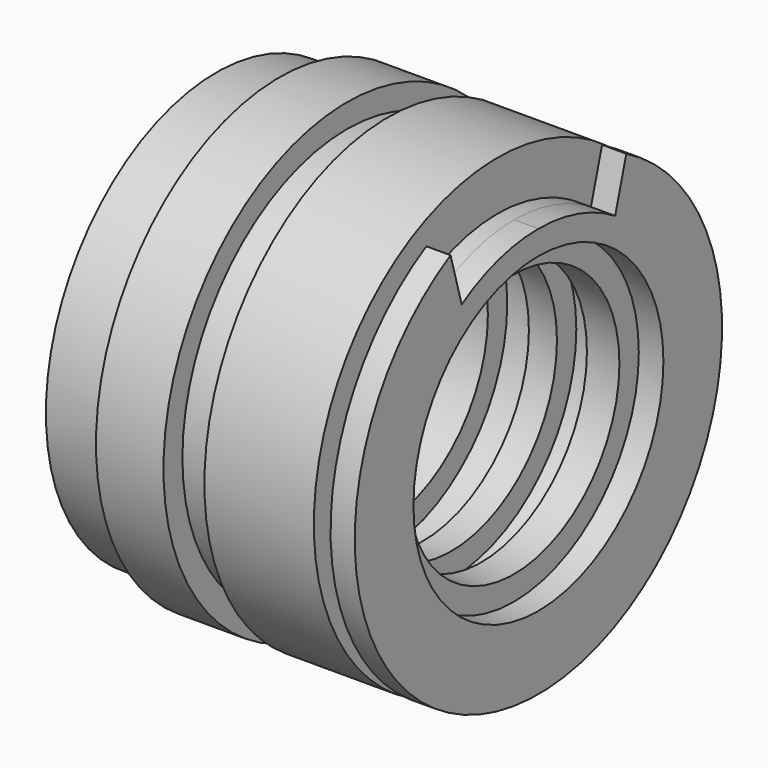
from build123d import *

# Parameters (mm, degrees)
F3_DEPTH = 4.6736


# Not quite as in the source:
# - after a boolean that leaves OpenCascade's solid faulty, fix() repairs it


with BuildPart() as f1:
    # F0 (on Top) → F1 (revolve)
    with BuildSketch(Plane.XY):
        Polygon((-4.7498, 30.1625), (0, 30.1625), (0, 44.323), (-4.6736, 44.323), (-4.6736, 34.798), (-7.8994, 34.798), (-7.8994, 44.323), (-29.0322, 44.323), (-29.0322, 39.751), (-36.9316, 39.751), (-36.9316, 44.323), (-49.9618, 44.323), (-49.9618, 41.1734), (-62.1538, 41.1734), (-62.1538, 25.4889), (-52.6288, 25.4889), (-52.6288, 28.575), (-39.9288, 28.575), (-39.9288, 25.4889), (-30.1498, 25.4889), (-30.1498, 30.1625), (-22.225, 30.1625), (-22.225, 25.4889), (-16.8148, 25.4889), (-16.8148, 30.1625), (-11.0236, 30.1625), (-11.0236, 25.4889), (-4.7498, 25.4889), align=None)
    revolve(axis=Axis((-31.0769, 0, 0), (-1, 0, 0)))

    # F2 (on face) → F3 (cut)
    with BuildSketch(Plane.YZ):
        with BuildLine():
            ThreePointArc((-18.5166, 29.4624562527), (-9.6349948448, 33.4375190219), (0, 34.798))
            Line((0, 34.798), (0, 44.323))
            ThreePointArc((0, 44.323), (-10.9432900176, 42.950817601), (-21.209, 38.9192323665))
            Line((-21.209, 38.9192323665), (-18.5166, 29.4624562527))
        make_face()
        with BuildLine():
            Line((0, 44.323), (0, 34.798))
            ThreePointArc((0, 34.798), (9.6349948448, 33.4375190219), (18.5166, 29.4624562527))
            Line((18.5166, 29.4624562527), (21.209, 38.9192323665))
            ThreePointArc((21.209, 38.9192323665), (10.9432900176, 42.950817601), (0, 44.323))
        make_face()
    extrude(amount=-F3_DEPTH, mode=Mode.SUBTRACT)

    add(f1.part.fix(), mode=Mode.REPLACE)


solid = f1.part
